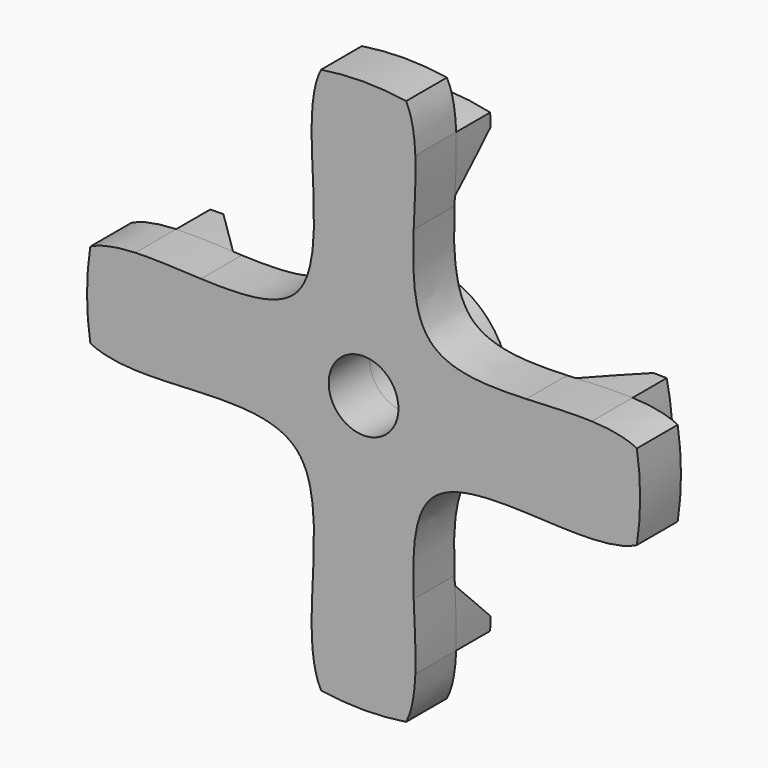
from build123d import *

# Parameters (mm, degrees)
F0_R         = 10
F0_R_2       = 4.1
F1_DEPTH     = 6
F2_DEPTH     = 5
F3_T4_ANGLE  = 122.6619234407
F3_T9_ANGLE  = 122.6619234407
F3_T14_ANGLE = 122.6619234407
F3_T19_ANGLE = 122.6619234407
F4_DEPTH     = 3


# Not quite as in the source:
# - a fillet or chamfer that OpenCascade refuses, or shapes differently, is made with other operations: its cross-section is extruded or revolved along the edge and cut away or added


with BuildPart() as f1:
    # F0 (on Front) → F1 (new body)
    with BuildSketch(Plane.XZ):
        with BuildLine():
            ThreePointArc((6.0812075174, 26.8191893079), (0, 27.5), (-6.0812075174, 26.8191893079))
            add(Edge.make_bspline(
                [(-6.0812075174, 26.8191893079), (-6.1732948606, 24.4249400285), (-5.9896734895, 21.7342705806), (-5.8889521452, 19.1133524697)],
                knots=[0.1196507891, 0.1196507891, 0.1196507891, 0.1196507891, 0.2585348809, 0.2585348809, 0.2585348809, 0.2585348809], degree=3))
            ThreePointArc((-5.8889521452, 19.1133524697), (0, 20), (5.8889521452, 19.1133524697))
            add(Edge.make_bspline(
                [(6.0812075174, 26.8191893079), (6.1732948606, 24.4249400285), (5.9896734895, 21.7342705806), (5.8889521452, 19.1133524697)],
                knots=[0.1196507891, 0.1196507891, 0.1196507891, 0.1196507891, 0.2585348809, 0.2585348809, 0.2585348809, 0.2585348809], degree=3))
        make_face()
        with BuildLine():
            add(Edge.make_bspline(
                [(26.8191893079, 6.0812075174), (28.8818720221, 6.0018728496), (30.7245490644, 5.7179047345), (32.1130814467, 5)],
                knots=[0.8803492109, 0.8803492109, 0.8803492109, 0.8803492109, 1, 1, 1, 1], degree=3))
            ThreePointArc((26.8191893079, 6.0812075174), (27.3292673334, 3.0595991595), (27.5, 0))
            ThreePointArc((27.5, 0), (27.3292673334, -3.0595991595), (26.8191893079, -6.0812075174))
            add(Edge.make_bspline(
                [(26.8191893079, -6.0812075174), (28.8818720221, -6.0018728496), (30.7245490644, -5.7179047345), (32.1130814467, -5)],
                knots=[0.8803492109, 0.8803492109, 0.8803492109, 0.8803492109, 1, 1, 1, 1], degree=3))
            ThreePointArc((32.1130814467, -5), (32.4031259836, -2.5074741258), (32.5, 0))
            ThreePointArc((32.5, 0), (32.4031259836, 2.5074741258), (32.1130814467, 5))
        make_face()
        with BuildLine():
            ThreePointArc((5, 32.1130814467), (0, 32.5), (-5, 32.1130814467))
            add(Edge.make_bspline(
                [(-5, 32.1130814467), (-5.7179047345, 30.7245490644), (-6.0018728496, 28.8818720221), (-6.0812075174, 26.8191893079)],
                knots=[0, 0, 0, 0, 0.1196507891, 0.1196507891, 0.1196507891, 0.1196507891], degree=3))
            ThreePointArc((-6.0812075174, 26.8191893079), (0, 27.5), (6.0812075174, 26.8191893079))
            add(Edge.make_bspline(
                [(5, 32.1130814467), (5.7179047345, 30.7245490644), (6.0018728496, 28.8818720221), (6.0812075174, 26.8191893079)],
                knots=[0, 0, 0, 0, 0.1196507891, 0.1196507891, 0.1196507891, 0.1196507891], degree=3))
        make_face()
        with BuildLine():
            add(Edge.make_bspline(
                [(-5, -32.1130814467), (-5.7179047345, -30.7245490644), (-6.0018728496, -28.8818720221), (-6.0812075174, -26.8191893079)],
                knots=[0, 0, 0, 0, 0.1196507891, 0.1196507891, 0.1196507891, 0.1196507891], degree=3))
            ThreePointArc((-5, -32.1130814467), (0, -32.5), (5, -32.1130814467))
            add(Edge.make_bspline(
                [(5, -32.1130814467), (5.7179047345, -30.7245490644), (6.0018728496, -28.8818720221), (6.0812075174, -26.8191893079)],
                knots=[0, 0, 0, 0, 0.1196507891, 0.1196507891, 0.1196507891, 0.1196507891], degree=3))
            ThreePointArc((6.0812075174, -26.8191893079), (0, -27.5), (-6.0812075174, -26.8191893079))
        make_face()
        with BuildLine():
            add(Edge.make_bspline(
                [(-26.8191893079, 6.0812075174), (-28.8818720221, 6.0018728496), (-30.7245490644, 5.7179047345), (-32.1130814467, 5)],
                knots=[0.8803492109, 0.8803492109, 0.8803492109, 0.8803492109, 1, 1, 1, 1], degree=3))
            ThreePointArc((-32.1130814467, 5), (-32.5, 0), (-32.1130814467, -5))
            add(Edge.make_bspline(
                [(-26.8191893079, -6.0812075174), (-28.8818720221, -6.0018728496), (-30.7245490644, -5.7179047345), (-32.1130814467, -5)],
                knots=[0.8803492109, 0.8803492109, 0.8803492109, 0.8803492109, 1, 1, 1, 1], degree=3))
            ThreePointArc((-26.8191893079, -6.0812075174), (-27.5, 0), (-26.8191893079, 6.0812075174))
        make_face()
        with BuildLine():
            add(Edge.make_bspline(
                [(-5.8889521452, 19.1133524697), (-5.713837119, 14.556600899), (-5.864780991, 5.864780991), (-14.556600899, 5.713837119), (-19.1133524697, 5.8889521452)],
                knots=[0.2585348809, 0.2585348809, 0.2585348809, 0.2585348809, 0.5, 0.7414651191, 0.7414651191, 0.7414651191, 0.7414651191], degree=3))
            ThreePointArc((-19.1133524697, 5.8889521452), (-20, 0), (-19.1133524697, -5.8889521452))
            add(Edge.make_bspline(
                [(-5.8889521452, -19.1133524697), (-5.713837119, -14.556600899), (-5.864780991, -5.864780991), (-14.556600899, -5.713837119), (-19.1133524697, -5.8889521452)],
                knots=[0.2585348809, 0.2585348809, 0.2585348809, 0.2585348809, 0.5, 0.7414651191, 0.7414651191, 0.7414651191, 0.7414651191], degree=3))
            ThreePointArc((-5.8889521452, -19.1133524697), (0, -20), (5.8889521452, -19.1133524697))
            add(Edge.make_bspline(
                [(5.8889521452, -19.1133524697), (5.713837119, -14.556600899), (5.864780991, -5.864780991), (14.556600899, -5.713837119), (19.1133524697, -5.8889521452)],
                knots=[0.2585348809, 0.2585348809, 0.2585348809, 0.2585348809, 0.5, 0.7414651191, 0.7414651191, 0.7414651191, 0.7414651191], degree=3))
            ThreePointArc((19.1133524697, -5.8889521452), (19.7770959622, -2.9776627248), (20, 0))
            ThreePointArc((20, 0), (19.7770959622, 2.9776627248), (19.1133524697, 5.8889521452))
            add(Edge.make_bspline(
                [(5.8889521452, 19.1133524697), (5.713837119, 14.556600899), (5.864780991, 5.864780991), (14.556600899, 5.713837119), (19.1133524697, 5.8889521452)],
                knots=[0.2585348809, 0.2585348809, 0.2585348809, 0.2585348809, 0.5, 0.7414651191, 0.7414651191, 0.7414651191, 0.7414651191], degree=3))
            ThreePointArc((5.8889521452, 19.1133524697), (0, 20), (-5.8889521452, 19.1133524697))
        make_face()
        Circle(F0_R, mode=Mode.SUBTRACT)
        with BuildLine():
            add(Edge.make_bspline(
                [(-6.0812075174, -26.8191893079), (-6.1732948606, -24.4249400285), (-5.9896734895, -21.7342705806), (-5.8889521452, -19.1133524697)],
                knots=[0.1196507891, 0.1196507891, 0.1196507891, 0.1196507891, 0.2585348809, 0.2585348809, 0.2585348809, 0.2585348809], degree=3))
            ThreePointArc((-6.0812075174, -26.8191893079), (0, -27.5), (6.0812075174, -26.8191893079))
            add(Edge.make_bspline(
                [(6.0812075174, -26.8191893079), (6.1732948606, -24.4249400285), (5.9896734895, -21.7342705806), (5.8889521452, -19.1133524697)],
                knots=[0.1196507891, 0.1196507891, 0.1196507891, 0.1196507891, 0.2585348809, 0.2585348809, 0.2585348809, 0.2585348809], degree=3))
            ThreePointArc((5.8889521452, -19.1133524697), (0, -20), (-5.8889521452, -19.1133524697))
        make_face()
        with BuildLine():
            ThreePointArc((27.5, 0), (27.3292673334, 3.0595991595), (26.8191893079, 6.0812075174))
            add(Edge.make_bspline(
                [(19.1133524697, 5.8889521452), (21.7342705806, 5.9896734895), (24.4249400285, 6.1732948606), (26.8191893079, 6.0812075174)],
                knots=[0.7414651191, 0.7414651191, 0.7414651191, 0.7414651191, 0.8803492109, 0.8803492109, 0.8803492109, 0.8803492109], degree=3))
            ThreePointArc((19.1133524697, 5.8889521452), (19.7770959622, 2.9776627248), (20, 0))
            ThreePointArc((20, 0), (19.7770959622, -2.9776627248), (19.1133524697, -5.8889521452))
            add(Edge.make_bspline(
                [(19.1133524697, -5.8889521452), (21.7342705806, -5.9896734895), (24.4249400285, -6.1732948606), (26.8191893079, -6.0812075174)],
                knots=[0.7414651191, 0.7414651191, 0.7414651191, 0.7414651191, 0.8803492109, 0.8803492109, 0.8803492109, 0.8803492109], degree=3))
            ThreePointArc((26.8191893079, -6.0812075174), (27.3292673334, -3.0595991595), (27.5, 0))
        make_face()
        with BuildLine():
            add(Edge.make_bspline(
                [(-19.1133524697, 5.8889521452), (-21.7342705806, 5.9896734895), (-24.4249400285, 6.1732948606), (-26.8191893079, 6.0812075174)],
                knots=[0.7414651191, 0.7414651191, 0.7414651191, 0.7414651191, 0.8803492109, 0.8803492109, 0.8803492109, 0.8803492109], degree=3))
            ThreePointArc((-26.8191893079, 6.0812075174), (-27.5, 0), (-26.8191893079, -6.0812075174))
            add(Edge.make_bspline(
                [(-19.1133524697, -5.8889521452), (-21.7342705806, -5.9896734895), (-24.4249400285, -6.1732948606), (-26.8191893079, -6.0812075174)],
                knots=[0.7414651191, 0.7414651191, 0.7414651191, 0.7414651191, 0.8803492109, 0.8803492109, 0.8803492109, 0.8803492109], degree=3))
            ThreePointArc((-19.1133524697, -5.8889521452), (-20, 0), (-19.1133524697, 5.8889521452))
        make_face()
        Circle(F0_R)
        Circle(F0_R_2, mode=Mode.SUBTRACT)
    extrude(amount=F1_DEPTH)

    # F0 (on Front) → F2 (join)
    with BuildSketch(Plane.XZ):
        with BuildLine():
            ThreePointArc((6.0812075174, 26.8191893079), (0, 27.5), (-6.0812075174, 26.8191893079))
            add(Edge.make_bspline(
                [(-6.0812075174, 26.8191893079), (-6.1732948606, 24.4249400285), (-5.9896734895, 21.7342705806), (-5.8889521452, 19.1133524697)],
                knots=[0.1196507891, 0.1196507891, 0.1196507891, 0.1196507891, 0.2585348809, 0.2585348809, 0.2585348809, 0.2585348809], degree=3))
            ThreePointArc((-5.8889521452, 19.1133524697), (0, 20), (5.8889521452, 19.1133524697))
            add(Edge.make_bspline(
                [(6.0812075174, 26.8191893079), (6.1732948606, 24.4249400285), (5.9896734895, 21.7342705806), (5.8889521452, 19.1133524697)],
                knots=[0.1196507891, 0.1196507891, 0.1196507891, 0.1196507891, 0.2585348809, 0.2585348809, 0.2585348809, 0.2585348809], degree=3))
        make_face()
        with BuildLine():
            ThreePointArc((27.5, 0), (27.3292673334, 3.0595991595), (26.8191893079, 6.0812075174))
            add(Edge.make_bspline(
                [(19.1133524697, 5.8889521452), (21.7342705806, 5.9896734895), (24.4249400285, 6.1732948606), (26.8191893079, 6.0812075174)],
                knots=[0.7414651191, 0.7414651191, 0.7414651191, 0.7414651191, 0.8803492109, 0.8803492109, 0.8803492109, 0.8803492109], degree=3))
            ThreePointArc((19.1133524697, 5.8889521452), (19.7770959622, 2.9776627248), (20, 0))
            ThreePointArc((20, 0), (19.7770959622, -2.9776627248), (19.1133524697, -5.8889521452))
            add(Edge.make_bspline(
                [(19.1133524697, -5.8889521452), (21.7342705806, -5.9896734895), (24.4249400285, -6.1732948606), (26.8191893079, -6.0812075174)],
                knots=[0.7414651191, 0.7414651191, 0.7414651191, 0.7414651191, 0.8803492109, 0.8803492109, 0.8803492109, 0.8803492109], degree=3))
            ThreePointArc((26.8191893079, -6.0812075174), (27.3292673334, -3.0595991595), (27.5, 0))
        make_face()
        with BuildLine():
            add(Edge.make_bspline(
                [(-19.1133524697, 5.8889521452), (-21.7342705806, 5.9896734895), (-24.4249400285, 6.1732948606), (-26.8191893079, 6.0812075174)],
                knots=[0.7414651191, 0.7414651191, 0.7414651191, 0.7414651191, 0.8803492109, 0.8803492109, 0.8803492109, 0.8803492109], degree=3))
            ThreePointArc((-26.8191893079, 6.0812075174), (-27.5, 0), (-26.8191893079, -6.0812075174))
            add(Edge.make_bspline(
                [(-19.1133524697, -5.8889521452), (-21.7342705806, -5.9896734895), (-24.4249400285, -6.1732948606), (-26.8191893079, -6.0812075174)],
                knots=[0.7414651191, 0.7414651191, 0.7414651191, 0.7414651191, 0.8803492109, 0.8803492109, 0.8803492109, 0.8803492109], degree=3))
            ThreePointArc((-19.1133524697, -5.8889521452), (-20, 0), (-19.1133524697, 5.8889521452))
        make_face()
        with BuildLine():
            add(Edge.make_bspline(
                [(-6.0812075174, -26.8191893079), (-6.1732948606, -24.4249400285), (-5.9896734895, -21.7342705806), (-5.8889521452, -19.1133524697)],
                knots=[0.1196507891, 0.1196507891, 0.1196507891, 0.1196507891, 0.2585348809, 0.2585348809, 0.2585348809, 0.2585348809], degree=3))
            ThreePointArc((-6.0812075174, -26.8191893079), (0, -27.5), (6.0812075174, -26.8191893079))
            add(Edge.make_bspline(
                [(6.0812075174, -26.8191893079), (6.1732948606, -24.4249400285), (5.9896734895, -21.7342705806), (5.8889521452, -19.1133524697)],
                knots=[0.1196507891, 0.1196507891, 0.1196507891, 0.1196507891, 0.2585348809, 0.2585348809, 0.2585348809, 0.2585348809], degree=3))
            ThreePointArc((5.8889521452, -19.1133524697), (0, -20), (-5.8889521452, -19.1133524697))
        make_face()
    extrude(amount=-F2_DEPTH)

    # F3: chamfer of 6 on 4 edges, made by hand


with BuildPart() as f3_tool2:
    # F3_s3 → F3_t4 (revolve)
    with BuildSketch(Plane(origin=(0, 0, 0), x_dir=(0, 1, 0), z_dir=(-0.4797494316, 0, -0.8774055407))):
        Polygon((-1, -20), (5, -26), (5, -20), align=None)
    revolve(axis=Axis((0, 5, 0), (0, 1, 0)), revolution_arc=F3_T4_ANGLE)

    split(bisect_by=Plane.XZ, keep=Keep.BOTTOM)


with BuildPart() as f1_1:
    add(f1.part)

    # F3_t1: cut F3_tool2
    add(f3_tool2.part, mode=Mode.SUBTRACT)


with BuildPart() as f3_tool7:
    # F3_s8 → F3_t9 (revolve)
    with BuildSketch(Plane(origin=(0, 0, 0), x_dir=(0, 1, 0), z_dir=(-0.8774055407, 0, 0.4797494316))):
        Polygon((-1, -20), (5, -26), (5, -20), align=None)
    revolve(axis=Axis((0, 5, 0), (0, 1, 0)), revolution_arc=F3_T9_ANGLE)

    split(bisect_by=Plane.XZ, keep=Keep.BOTTOM)


with BuildPart() as f1_2:
    add(f1_1.part)

    # F3_t6: cut F3_tool7
    add(f3_tool7.part, mode=Mode.SUBTRACT)


with BuildPart() as f3_tool12:
    # F3_s13 → F3_t14 (revolve)
    with BuildSketch(Plane(origin=(0, 0, 0), x_dir=(0, 1, 0), z_dir=(0.8774055407, 0, -0.4797494316))):
        Polygon((-1, -20), (5, -26), (5, -20), align=None)
    revolve(axis=Axis((0, 5, 0), (0, 1, 0)), revolution_arc=F3_T14_ANGLE)

    split(bisect_by=Plane.XZ, keep=Keep.BOTTOM)


with BuildPart() as f1_3:
    add(f1_2.part)

    # F3_t11: cut F3_tool12
    add(f3_tool12.part, mode=Mode.SUBTRACT)


with BuildPart() as f3_tool17:
    # F3_s18 → F3_t19 (revolve)
    with BuildSketch(Plane(origin=(0, 0, 0), x_dir=(0, 1, 0), z_dir=(0.4797494316, 0, 0.8774055407))):
        Polygon((-1, -20), (5, -26), (5, -20), align=None)
    revolve(axis=Axis((0, 5, 0), (0, 1, 0)), revolution_arc=F3_T19_ANGLE)

    split(bisect_by=Plane.XZ, keep=Keep.BOTTOM)


with BuildPart() as f1_4:
    add(f1_3.part)

    # F3_t16: cut F3_tool17
    add(f3_tool17.part, mode=Mode.SUBTRACT)

    # F0 (on Front) → F4 (join)
    with BuildSketch(Plane.XZ):
        Circle(F0_R)
        Circle(F0_R_2, mode=Mode.SUBTRACT)
    extrude(amount=-F4_DEPTH)


solid = f1_4.part
